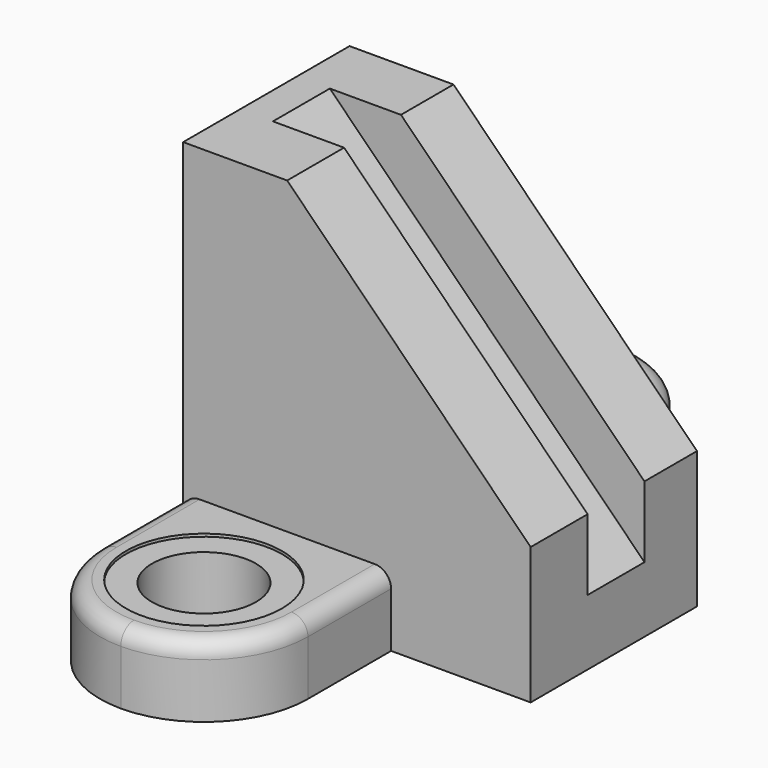
from build123d import *

# Parameters (mm, degrees)
F0_W      = 127
F0_H      = 76
F1_DEPTH  = 200
F3_DEPTH  = 76.001
F4_W      = 26
F4_H      = 26
F6_W      = 76
F6_H      = 26
F7_DEPTH  = 76
F8_R      = 37.99999
F9_W      = 76
F9_H      = 26
F10_DEPTH = 76
F11_R     = 37.99999
F12_R     = 19
F13_DEPTH = 26.001
F12_R_2   = 28.5
F14_DEPTH = 1
F15_R     = 6
F16_R     = 28.5
F16_R_2   = 19
F17_DEPTH = 1
F18_DEPTH = 26


# Not quite as in the source:
# - a fillet or chamfer is up to 0.001 mm smaller than in the source, because OpenCascade refuses the exact size
# - a feature names something its author has since deleted; it is built from what else it names


with BuildPart() as f1:
    # F0 (on Top) → F1 (new body)
    with BuildSketch(Plane.XY):
        with Locations((63.5, 38)):
            Rectangle(F0_W, F0_H)
    extrude(amount=F1_DEPTH)

    # F2 (on face) → F3 (cut, through all)
    with BuildSketch(Plane.XZ):
        Polygon((38, 139), (127, 50), (127, 200), (0, 200), (0, 177), align=None)
        Polygon((0, 139), (38, 139), (0, 177), align=None)
    extrude(amount=-F3_DEPTH, mode=Mode.SUBTRACT)

    # F5: sweep along a path in F2
    with BuildLine(Plane.XZ) as f5_path:
        Line((0, 177), (191.2105315588, -14.2105315588))
    # F4 (on face) → F5 (sweep, cut)
    with BuildSketch(Plane.XY.offset(139)):
        with Locations((25, 39)):
            Rectangle(F4_W, F4_H)
    sweep(path=f5_path.line, mode=Mode.SUBTRACT)

    # F6 (on face) → F7 (join)
    with BuildSketch(Plane.XZ):
        with Locations((38, 13)):
            Rectangle(F6_W, F6_H)
    extrude(amount=F7_DEPTH)

    # F8 (radius 38 in the source; OpenCascade refuses exactly that, so slightly less here)
    f8_edges = [f1.edges().sort_by_distance(p)[0] for p in [
        (76, -76, 13),
        (0, -76, 13),
    ]]
    fillet(f8_edges, radius=F8_R)

    # F9 (on face) → F10 (join)
    with BuildSketch(Plane(origin=(0, 76, 0), x_dir=(-1, 0, 0), z_dir=(0, 1, 0))):
        with Locations((-38, 13)):
            Rectangle(F9_W, F9_H)
    extrude(amount=F10_DEPTH)

    # F11 (radius 38 in the source; OpenCascade refuses exactly that, so slightly less here)
    f11_edges = [f1.edges().sort_by_distance(p)[0] for p in [
        (0, 152, 13),
        (76, 152, 13),
    ]]
    fillet(f11_edges, radius=F11_R)

    # F12 (on face) → F13 (cut, through all)
    with BuildSketch(Plane.XY.offset(26)):
        with Locations((38, 114)):
            Circle(F12_R)
    extrude(amount=-F13_DEPTH, mode=Mode.SUBTRACT)

    # F12 (on face) → F14 (cut)
    with BuildSketch(Plane.XY.offset(26)):
        with Locations((38, 114)):
            Circle(F12_R_2)
        with Locations((38, 114)):
            Circle(F12_R, mode=Mode.SUBTRACT)
    extrude(amount=-F14_DEPTH, mode=Mode.SUBTRACT)

    # F15
    f15_edges = [f1.edges().sort_by_distance(p)[0] for p in [
        (64.870061, 140.870061, 26),
        (11.129939, -64.870061, 26),
    ]]
    fillet(f15_edges, radius=F15_R)

    # F16 (on face) → F17 (cut)
    with BuildSketch(Plane.XY.offset(26)):
        with Locations((38, -38)):
            Circle(F16_R)
        with Locations((38, -38)):
            Circle(F16_R_2, mode=Mode.SUBTRACT)
    extrude(amount=-F17_DEPTH, mode=Mode.SUBTRACT)

    # F18 (cut, through all): a face of the model
    f18_faces = [f1.faces().sort_by_distance(p)[0] for p in [
        (38, -38, 26),
    ]]
    extrude(f18_faces, amount=-F18_DEPTH, mode=Mode.SUBTRACT)


solid = f1.part
